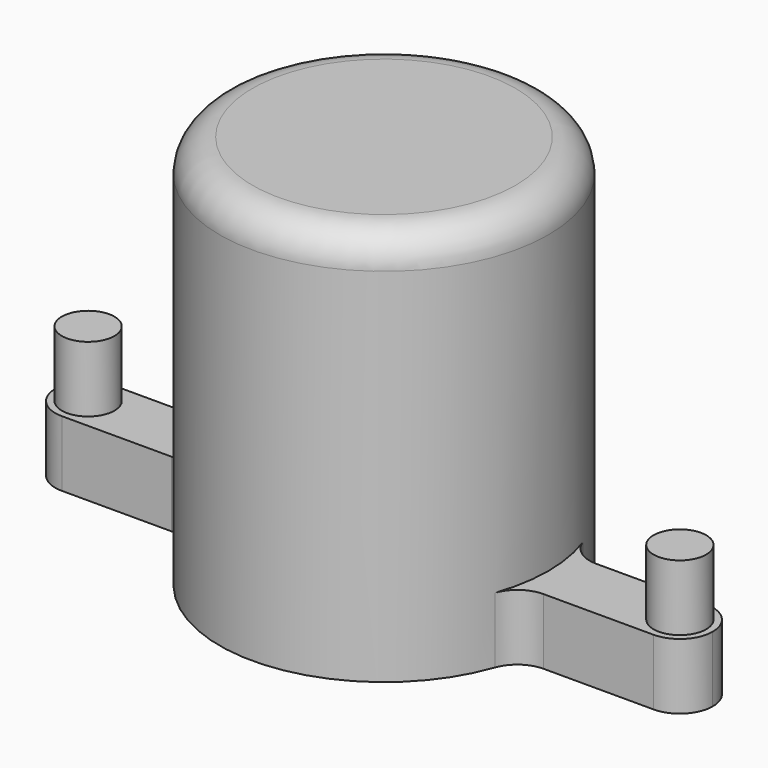
from build123d import *

# Parameters (mm, degrees)
F0_R      = 25
F1_DEPTH  = 50
F2_R      = 5
F3_W      = 100
F3_H      = 10
F4_DEPTH  = 10
F5_R      = 4.99999
F6_R      = 4
F7_DEPTH  = 10
F8_DEPTH  = 10
F10_DEPTH = 40
F11_R     = 5


# Not quite as in the source:
# - a fillet or chamfer is up to 0.001 mm smaller than in the source, because OpenCascade refuses the exact size


with BuildPart() as f1:
    # F0 (on Top) → F1 (new body)
    with BuildSketch(Plane.XY):
        Circle(F0_R)
    extrude(amount=F1_DEPTH)

    # F2
    f2_edges = [f1.edges().sort_by_distance(p)[0] for p in [
        (-25, 0, 50),
    ]]
    fillet(f2_edges, radius=F2_R)

    # F3 (on face) → F4 (join)
    with BuildSketch(Plane(origin=(0, 0, 0), x_dir=(1, 0, 0), z_dir=(0, 0, -1))):
        Rectangle(F3_W, F3_H)
    extrude(amount=F4_DEPTH)

    # F5 (radius 5 in the source; OpenCascade refuses exactly that, so slightly less here)
    f5_edges = [f1.edges().sort_by_distance(p)[0] for p in [
        (-50, 5, -5),
        (-50, -5, -5),
        (50, -5, -5),
        (50, 5, -5),
    ]]
    fillet(f5_edges, radius=F5_R)

    # F6 (on face) → F7 (join)
    with BuildSketch(Plane.XY):
        with Locations((-45, 0)):
            Circle(F6_R)
        with Locations((45, 0)):
            Circle(F6_R)
    extrude(amount=F7_DEPTH)

    # F8 (add): faces of the model
    f8_faces = [f1.faces().sort_by_distance(p)[0] for p in [
        (0, -13.3591920493, 0),
        (0, 13.3591920493, 0),
    ]]
    extrude(f8_faces, amount=F8_DEPTH)

    # F9 (on face) → F10 (cut)
    with BuildSketch(Plane(origin=(0, 0, -10), x_dir=(1, 0, 0), z_dir=(0, 0, -1))):
        Polygon((1.575, 2.7279800219), (-1.575, 2.7279800219), (-3.15, 0), (-1.575, -2.7279800219), (1.575, -2.7279800219), (3.15, 0), align=None)
    extrude(amount=-F10_DEPTH, mode=Mode.SUBTRACT)

    # F11
    f11_edges = [f1.edges().sort_by_distance(p)[0] for p in [
        (23.535534, 0, 48.535534),
        (-25, 0, 45),
        (-20, 0, 50),
        (24.494897, 5, -5),
        (24.494897, -5, -5),
        (-24.494897, -5, -5),
        (-24.494897, 5, -5),
    ]]
    fillet(f11_edges, radius=F11_R)


solid = f1.part
